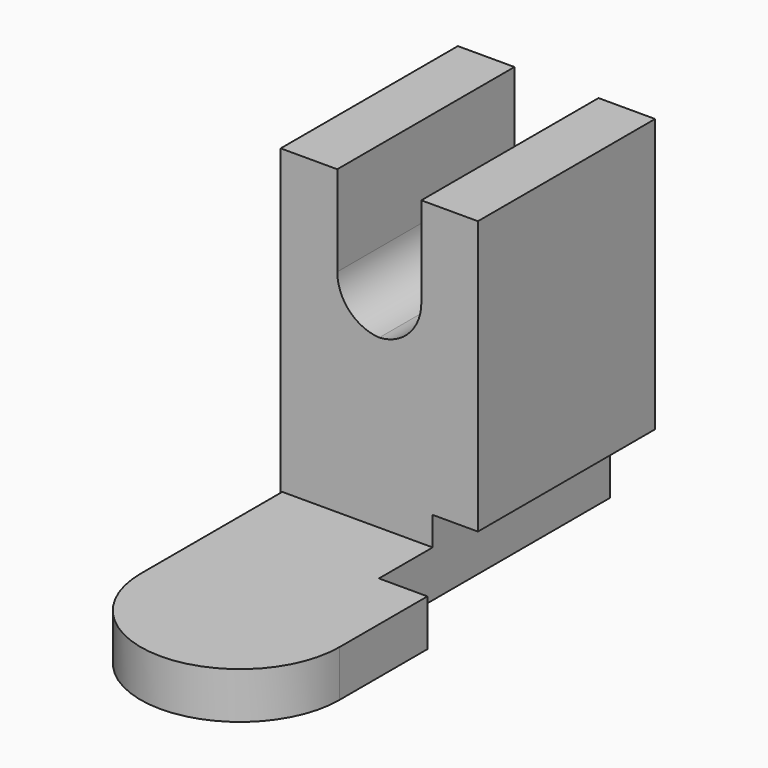
from build123d import *

# Parameters (mm, degrees)
F0_W        = 22.621599026
F0_H        = 39.9586446583
F1_DEPTH    = 25.4
F2_W        = 9.6419928595
F2_H        = 15.4364593327
F3_DEPTH    = 25.401
F4_T1_DEPTH = 25.4
F5_W        = 5.1918416284
F5_H        = 8.622167632
F6_DEPTH    = 25.401
F8_DEPTH    = 0.254
F9_DEPTH    = 5.08


# Not quite as in the source:
# - a fillet or chamfer that OpenCascade refuses, or shapes differently, is made with other operations: its cross-section is extruded or revolved along the edge and cut away or added


with BuildPart() as f1:
    # F0 (on Front) → F1 (new body)
    with BuildSketch(Plane.XZ):
        with Locations((0.185423065, 19.9793223292)):
            Rectangle(F0_W, F0_H)
    extrude(amount=F1_DEPTH)

    # F2 (on face) → F3 (cut, through all)
    with BuildSketch(Plane.XZ.offset(25.4)):
        with Locations((0.1854221337, 32.240414992)):
            Rectangle(F2_W, F2_H)
    extrude(amount=-F3_DEPTH, mode=Mode.SUBTRACT)

    # F4: fillet of radius 5.08 on 2 edges, made by hand

    # F4_s2 → F4_t1 (join)
    with BuildSketch(Plane.XZ):
        with BuildLine():
            ThreePointArc((-4.6355742961, 29.6021853256), (-3.1476767445, 26.0100828772), (0.4444257039, 24.5221853256))
            Line((0.4444257039, 24.5221853256), (-4.6355742961, 24.5221853256))
            Line((-4.6355742961, 24.5221853256), (-4.6355742961, 29.6021853256))
        make_face()
        with BuildLine():
            ThreePointArc((-0.0735814366, 24.5221853256), (3.5185210119, 26.0100828772), (5.0064185634, 29.6021853256))
            Line((5.0064185634, 29.6021853256), (5.0064185634, 24.5221853256))
            Line((5.0064185634, 24.5221853256), (-0.0735814366, 24.5221853256))
        make_face()
    extrude(amount=F4_T1_DEPTH)

    # F5 (on face) → F6 (cut, through all)
    with BuildSketch(Plane.XZ.offset(25.4)):
        with Locations((8.9003017638, 4.311083816)):
            Rectangle(F5_W, F5_H)
    extrude(amount=-F6_DEPTH, mode=Mode.SUBTRACT)

    # F7 (on Top) → F8 (join)
    with BuildSketch(Plane.XY):
        with BuildLine():
            Line((6.3043809496, 0), (-10.9399538487, 0))
            Line((-10.9399538487, 0), (-10.9399538487, -45.7067526877))
            ThreePointArc((-10.9399538487, -45.7067526877), (0.463556964, -57.1102635004), (11.8670677766, -45.7067526877))
            Line((11.8670677766, -45.7067526877), (11.8670677766, -33.1019833684))
            Line((11.8670677766, -33.1019833684), (6.3043809496, -33.1019833684))
            Line((6.3043809496, -33.1019833684), (6.3043809496, -25.4))
            Line((6.3043809496, -25.4), (6.3043809496, 0))
        make_face()
    extrude(amount=F8_DEPTH)

    # F9 (add): a face of the model
    f9_faces = [f1.faces().sort_by_distance(p)[0] for p in [
        (-0.1279092973, -40.8893319154, 0.254),
    ]]
    extrude(f9_faces, amount=F9_DEPTH)


solid = f1.part
